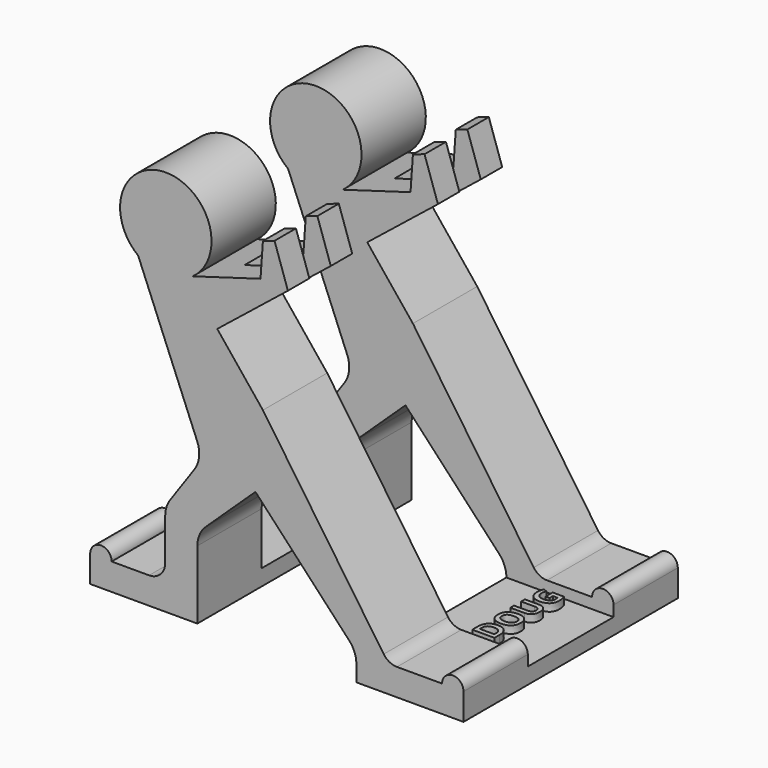
from build123d import *

# Parameters (mm, degrees)
F1_DEPTH      = 50
F2_R          = 3
F3_R          = 5
F4_W          = 20
F4_H          = 84.3465569907
F5_DEPTH      = 82.2
F6_W          = 5
F6_H          = 7.8074337992
F6_H_2        = 14.7454175439
F7_DEPTH      = 12
F8_W          = 5
F8_H          = 13.8043484801
F8_H_2        = 7.8074337992
F9_DEPTH      = 12
F10_R         = 3
F11_TEXT_SIZE = 5.7921366359
F12_DEPTH     = 1.4


# Not quite as in the source:
# - Text() gives the source's letters only with a copy of the font that has no kerning and outlines rounded to 1/6400 em; it was checked with that copy


with BuildPart() as f1:
    # F0 (on Front) → F1 (new body)
    with BuildSketch(Plane.XZ):
        with BuildLine():
            Line((72.3966664672, 5), (62.3966664672, 5))
            Line((62.3966664672, 5), (38.9506465123, 39.0608766391))
            Line((38.9506465123, 39.0608766391), (30.4268324003, 49.6403474958))
            Line((30.4268324003, 49.6403474958), (43.6172244836, 60.1968737297))
            Line((43.6172244836, 60.1968737297), (41.1178078351, 67.5934228539))
            Line((41.1178078351, 67.5934228539), (38.9506465123, 66.8611030924))
            Line((38.9506465123, 66.8611030924), (38.5009124875, 60.5004653335))
            Line((38.5009124875, 60.5004653335), (25.8558781635, 56.7960041687))
            ThreePointArc((25.8558781635, 56.7960041687), (20.9080707236, 72.2254824581), (15.6591438064, 56.8958260704))
            Line((15.6591438064, 56.8958260704), (26.6889118579, 29.9428857566))
            ThreePointArc((26.6889118579, 29.9428857566), (27.0334089022, 27.479718373), (26.1572763774, 25.1520019872))
            Line((26.1572763774, 25.1520019872), (20.7106787943, 17.3502100089))
            Line((20.7106787943, 17.3502100089), (20.7106787943, 5))
            Line((20.7106787943, 5), (10.7106787943, 5))
            ThreePointArc((10.7106787943, 5), (8.7106787943, 7), (6.7106787943, 5))
            Line((6.7106787943, 5), (6.7106787943, 0))
            Line((6.7106787943, 0), (26.7106787943, 0))
            Line((26.7106787943, 0), (26.7106787943, 14.9260010963))
            Line((26.7106787943, 14.9260010963), (37.5600930936, 25.1781505826))
            Line((37.5600930936, 25.1781505826), (56.3966664672, 5))
            Line((56.3966664672, 5), (56.3966664672, 0))
            Line((56.3966664672, 0), (76.3966664672, 0))
            Line((76.3966664672, 0), (76.3966664672, 5))
            ThreePointArc((76.3966664672, 5), (74.3966664672, 7), (72.3966664672, 5))
        make_face()
    extrude(amount=F1_DEPTH)

    # F2
    f2_edges = [f1.edges().sort_by_distance(p)[0] for p in [
        (20.710679, -25, 5),
    ]]
    fillet(f2_edges, radius=F2_R)

    # F3
    f3_edges = [f1.edges().sort_by_distance(p)[0] for p in [
        (56.396666, -25, 5),
        (26.710679, -25, 14.926001),
        (20.710679, -25, 17.35021),
    ]]
    fillet(f3_edges, radius=F3_R)

    # F4 (on Right) → F5 (cut)
    with BuildSketch(Plane.YZ):
        with Locations((-25, 45.1732784954)):
            Rectangle(F4_W, F4_H)
    extrude(amount=F5_DEPTH, mode=Mode.SUBTRACT)

    # F6 (on face) → F7 (cut)
    with BuildSketch(Plane(origin=(57.4039286604, 0, 19.397739753), x_dir=(0, 1, 0), z_dir=(0.9473726341, 0, 0.3201329288))):
        with Locations((-42.5, 46.969277912)):
            Rectangle(F6_W, F6_H)
        with Locations((-42.5, 35.6928522404)):
            Rectangle(F6_W, F6_H_2)
    extrude(amount=-F7_DEPTH, mode=Mode.SUBTRACT)

    # F8 (on face) → F9 (cut)
    with BuildSketch(Plane(origin=(57.4039286604, 0, 19.397739753), x_dir=(0, 1, 0), z_dir=(0.9473726341, 0, 0.3201329288))):
        with Locations((-7.5, 36.1633867723)):
            Rectangle(F8_W, F8_H)
        with Locations((-7.5, 46.969277912)):
            Rectangle(F8_W, F8_H_2)
    extrude(amount=-F9_DEPTH, mode=Mode.SUBTRACT)

    # F10
    f10_edges = [f1.edges().sort_by_distance(p)[0] for p in [
        (62.396666, -42.5, 5),
        (62.396666, -7.5, 5),
    ]]
    fillet(f10_edges, radius=F10_R)

    # F11 (on face) → F12 (join)
    with BuildSketch(Plane.XY.offset(3)):
        with Locations(Location((68.6179499482, -33.5827434361), (0, 0, 90))):
            Text('DOUG', F11_TEXT_SIZE, font='Open Sans', font_style=FontStyle.BOLD, text_align=(TextAlign.LEFT, TextAlign.BOTTOM))
    extrude(amount=F12_DEPTH)


solid = f1.part
